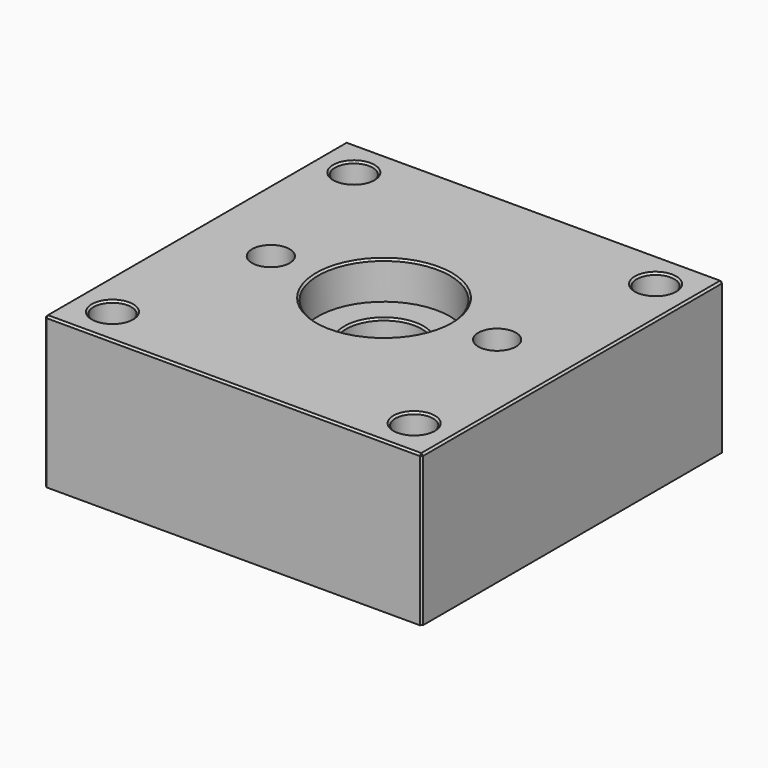
from build123d import *

# Parameters (mm, degrees)
F0_W     = 20
F0_H     = 20
F0_R     = 1
F0_R_2   = 8.5
F0_R_3   = 7
F0_R_4   = 6.5
F0_R_5   = 1.25
F0_R_6   = 2
F1_DEPTH = 8
F2_R     = 3.5
F2_R_2   = 2
F3_DEPTH = 2
F4_SIZE  = 0.1
F5_DEPTH = 4
F6_R     = 1
F7_DEPTH = 3


with BuildPart() as f1:
    # F0 (on Top) → F1 (new body)
    with BuildSketch(Plane.XY):
        with Locations((10, -10)):
            Rectangle(F0_W, F0_H)
        with Locations((2, -18)):
            Circle(F0_R, mode=Mode.SUBTRACT)
        with Locations((18, -18)):
            Circle(F0_R, mode=Mode.SUBTRACT)
        with Locations((2, -2)):
            Circle(F0_R, mode=Mode.SUBTRACT)
        with Locations((10, -10)):
            Circle(F0_R_2, mode=Mode.SUBTRACT)
        with Locations((18, -2)):
            Circle(F0_R, mode=Mode.SUBTRACT)
        with Locations((10, -10)):
            Circle(F0_R_2)
        with Locations((10, -10)):
            Circle(F0_R_3, mode=Mode.SUBTRACT)
        with Locations((10, -10)):
            Circle(F0_R_3)
        with Locations((10, -10)):
            Circle(F0_R_4, mode=Mode.SUBTRACT)
        with Locations((10, -10)):
            Circle(F0_R_4)
        with BuildLine():
            ThreePointArc((11.25, -14.25), (9.1161165153, -15.1338834682), (10.0000000233, -13))
            ThreePointArc((10.0000000233, -13), (10.8838834847, -13.3661165318), (11.25, -14.25))
        make_face(mode=Mode.SUBTRACT)
        with Locations((5.75, -10)):
            Circle(F0_R_5, mode=Mode.SUBTRACT)
        with BuildLine():
            ThreePointArc((10, -7), (12.1213203436, -7.8786796564), (13, -10))
            ThreePointArc((13, -10), (12.1213203518, -12.1213203353), (10.0000000233, -13))
            ThreePointArc((10.0000000233, -13), (7.8786796647, -12.1213203518), (7, -10))
            ThreePointArc((7, -10), (7.8786796564, -7.8786796564), (10, -7))
        make_face(mode=Mode.SUBTRACT)
        with BuildLine():
            ThreePointArc((15.5, -10), (14.25, -11.25), (13, -10))
            ThreePointArc((13, -10), (14.25, -8.75), (15.5, -10))
        make_face(mode=Mode.SUBTRACT)
        with BuildLine():
            ThreePointArc((11.25, -5.75), (10.8838834765, -6.6338834765), (10, -7))
            ThreePointArc((10, -7), (9.1161165235, -4.8661165235), (11.25, -5.75))
        make_face(mode=Mode.SUBTRACT)
        with BuildLine():
            ThreePointArc((10.0000000233, -13), (12.1213203518, -12.1213203353), (13, -10))
            ThreePointArc((13, -10), (12.1213203436, -7.8786796564), (10, -7))
            ThreePointArc((10, -7), (7.8786796564, -7.8786796564), (7, -10))
            ThreePointArc((7, -10), (7.8786796647, -12.1213203518), (10.0000000233, -13))
        make_face()
        with Locations((10, -10)):
            Circle(F0_R_6, mode=Mode.SUBTRACT)
        with BuildLine():
            ThreePointArc((15.5, -10), (14.25, -8.75), (13, -10))
            ThreePointArc((13, -10), (14.25, -11.25), (15.5, -10))
        make_face()
        with BuildLine():
            ThreePointArc((11.25, -5.75), (9.1161165235, -4.8661165235), (10, -7))
            ThreePointArc((10, -7), (10.8838834765, -6.6338834765), (11.25, -5.75))
        make_face()
        with Locations((5.75, -10)):
            Circle(F0_R_5)
        with BuildLine():
            ThreePointArc((11.25, -14.25), (10.8838834847, -13.3661165318), (10.0000000233, -13))
            ThreePointArc((10.0000000233, -13), (9.1161165153, -15.1338834682), (11.25, -14.25))
        make_face()
    extrude(amount=F1_DEPTH)

    # F2 (on face) → F3 (cut)
    with BuildSketch(Plane.XY.offset(8)):
        with Locations((10, -10)):
            Circle(F2_R)
        with Locations((10, -10)):
            Circle(F2_R_2, mode=Mode.SUBTRACT)
    extrude(amount=-F3_DEPTH, mode=Mode.SUBTRACT)

    # F4
    f4_edges = [f1.edges().sort_by_distance(p)[0] for p in [
        (10, 0, 8),
        (20, -10, 8),
        (0, -10, 8),
        (10, -20, 8),
        (1, -18, 8),
        (17, -18, 8),
        (1, -2, 8),
        (6.5, -10, 8),
        (17, -2, 8),
        (20, -20, 4),
        (20, 0, 4),
        (0, -20, 4),
        (0, 0, 4),
        (8, -10, 6),
    ]]
    chamfer(f4_edges, length=F4_SIZE)

    # F0 (on Top) → F5 (cut)
    with BuildSketch(Plane.XY):
        with Locations((10, -10)):
            Circle(F0_R_4)
        with BuildLine():
            ThreePointArc((11.25, -14.25), (9.1161165153, -15.1338834682), (10.0000000233, -13))
            ThreePointArc((10.0000000233, -13), (10.8838834847, -13.3661165318), (11.25, -14.25))
        make_face(mode=Mode.SUBTRACT)
        with Locations((5.75, -10)):
            Circle(F0_R_5, mode=Mode.SUBTRACT)
        with BuildLine():
            ThreePointArc((10, -7), (12.1213203436, -7.8786796564), (13, -10))
            ThreePointArc((13, -10), (12.1213203518, -12.1213203353), (10.0000000233, -13))
            ThreePointArc((10.0000000233, -13), (7.8786796647, -12.1213203518), (7, -10))
            ThreePointArc((7, -10), (7.8786796564, -7.8786796564), (10, -7))
        make_face(mode=Mode.SUBTRACT)
        with BuildLine():
            ThreePointArc((15.5, -10), (14.25, -11.25), (13, -10))
            ThreePointArc((13, -10), (14.25, -8.75), (15.5, -10))
        make_face(mode=Mode.SUBTRACT)
        with BuildLine():
            ThreePointArc((11.25, -5.75), (10.8838834765, -6.6338834765), (10, -7))
            ThreePointArc((10, -7), (9.1161165235, -4.8661165235), (11.25, -5.75))
        make_face(mode=Mode.SUBTRACT)
        with BuildLine():
            ThreePointArc((10.0000000233, -13), (12.1213203518, -12.1213203353), (13, -10))
            ThreePointArc((13, -10), (12.1213203436, -7.8786796564), (10, -7))
            ThreePointArc((10, -7), (7.8786796564, -7.8786796564), (7, -10))
            ThreePointArc((7, -10), (7.8786796647, -12.1213203518), (10.0000000233, -13))
        make_face()
        with Locations((10, -10)):
            Circle(F0_R_6, mode=Mode.SUBTRACT)
        with BuildLine():
            ThreePointArc((15.5, -10), (14.25, -8.75), (13, -10))
            ThreePointArc((13, -10), (14.25, -11.25), (15.5, -10))
        make_face()
        with BuildLine():
            ThreePointArc((11.25, -14.25), (10.8838834847, -13.3661165318), (10.0000000233, -13))
            ThreePointArc((10.0000000233, -13), (9.1161165153, -15.1338834682), (11.25, -14.25))
        make_face()
        with Locations((5.75, -10)):
            Circle(F0_R_5)
        with BuildLine():
            ThreePointArc((11.25, -5.75), (9.1161165235, -4.8661165235), (10, -7))
            ThreePointArc((10, -7), (10.8838834765, -6.6338834765), (11.25, -5.75))
        make_face()
    extrude(amount=F5_DEPTH, mode=Mode.SUBTRACT)

    # F6 (on face) → F7 (cut)
    with BuildSketch(Plane.XY.offset(8)):
        with Locations((4, -10)):
            Circle(F6_R)
        with Locations((16, -10)):
            Circle(F6_R)
    extrude(amount=-F7_DEPTH, mode=Mode.SUBTRACT)


solid = f1.part
